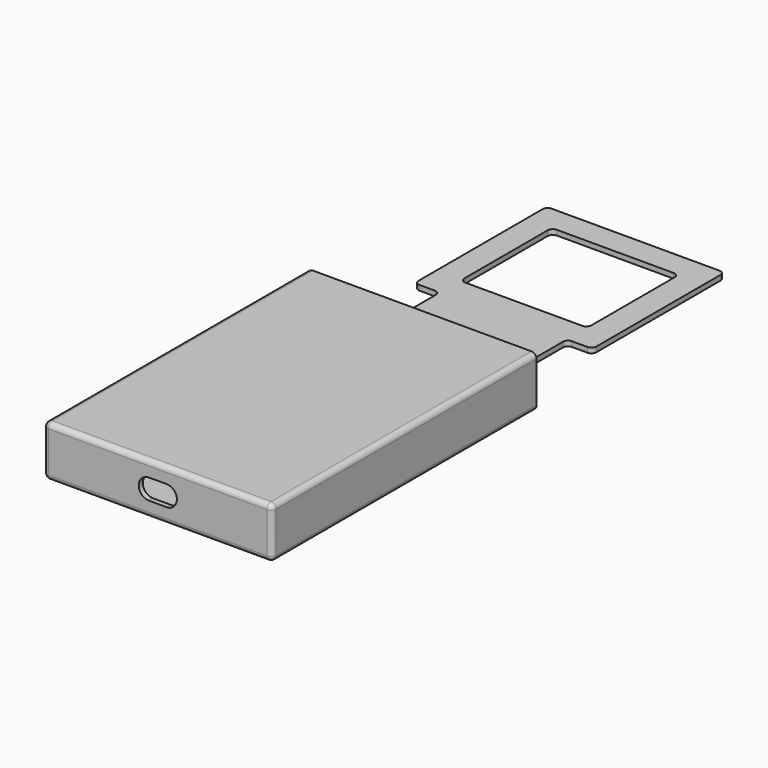
from build123d import *

# Parameters (mm, degrees)
F0_W      = 90
F0_H      = 130
F1_DEPTH  = 20
F2_W      = 50
F2_H      = 2
F3_DEPTH  = 40
F4_W      = 50
F4_H      = 45
F5_DEPTH  = 2
F6_T      = -2
F7_R      = 2
F8_R      = 2
F9_R      = 2
F10_R     = 2
F11_R     = 2
F13_DEPTH = 25


# Not quite as in the source:
# - a shell that OpenCascade refuses in one call is made with other operations: the cavity is built on its own and cut out


with BuildPart() as f1:
    # F0 (on Top) → F1 (new body)
    with BuildSketch(Plane.XY):
        with Locations((45, -65)):
            Rectangle(F0_W, F0_H)
    extrude(amount=F1_DEPTH)

    # F2 (on face) → F3 (join)
    with BuildSketch(Plane(origin=(0, 0, 0), x_dir=(-1, 0, 0), z_dir=(0, 1, 0))):
        with Locations((-45, 1)):
            Rectangle(F2_W, F2_H)
    extrude(amount=F3_DEPTH)

    # F4 (on Top) → F5 (join)
    with BuildSketch(Plane.XY):
        Polygon((20, 40), (70, 40), (80, 40), (80, 105), (10, 105), (10, 40), align=None)
        with Locations((45, 72.5)):
            Rectangle(F4_W, F4_H, mode=Mode.SUBTRACT)
    extrude(amount=F5_DEPTH)

    # F6: a shell. OpenCascade refuses it in one call, so the cavity is built on its own and cut out:
    # the body offset inwards by the wall thickness, plus a prism from it out through each open face.
    f6_core = offset(f1.part, amount=F6_T, kind=Kind.INTERSECTION, mode=Mode.PRIVATE)
    f6_exits = [f6_core.faces().sort_by_distance(p)[0] for p in [
        (45, -2, 10),
    ]]
    add(f6_core, mode=Mode.SUBTRACT)
    extrude(f6_exits, amount=-F6_T, mode=Mode.SUBTRACT)

    # F7
    f7_edges = [f1.edges().sort_by_distance(p)[0] for p in [
        (0, -65, 20),
        (90, -65, 20),
        (90, -65, 0),
        (0, -65, 0),
    ]]
    fillet(f7_edges, radius=F7_R)

    # F8
    f8_edges = [f1.edges().sort_by_distance(p)[0] for p in [
        (45, -130, 0),
    ]]
    fillet(f8_edges, radius=F8_R)

    # F9
    f9_edges = [f1.edges().sort_by_distance(p)[0] for p in [
        (10, 40, 1),
        (10, 105, 1),
        (80, 105, 1),
        (80, 40, 1),
    ]]
    fillet(f9_edges, radius=F9_R)

    # F10
    f10_edges = [f1.edges().sort_by_distance(p)[0] for p in [
        (20, 40, 1),
        (70, 40, 1),
        (70, 0, 1),
        (20, 0, 1),
    ]]
    fillet(f10_edges, radius=F10_R)

    # F11
    f11_edges = [f1.edges().sort_by_distance(p)[0] for p in [
        (20, 50, 1),
        (20, 95, 1),
        (70, 50, 1),
        (70, 95, 1),
    ]]
    fillet(f11_edges, radius=F11_R)

    # F12 (on face) → F13 (cut)
    with BuildSketch(Plane.XZ.offset(130)):
        with BuildLine():
            Line((48.5, 14), (41.5, 14))
            ThreePointArc((41.5, 14), (37.5, 10), (41.5, 6))
            Line((41.5, 6), (48.5, 6))
            ThreePointArc((48.5, 6), (52.5, 10), (48.5, 14))
        make_face()
    extrude(amount=-F13_DEPTH, mode=Mode.SUBTRACT)


solid = f1.part
